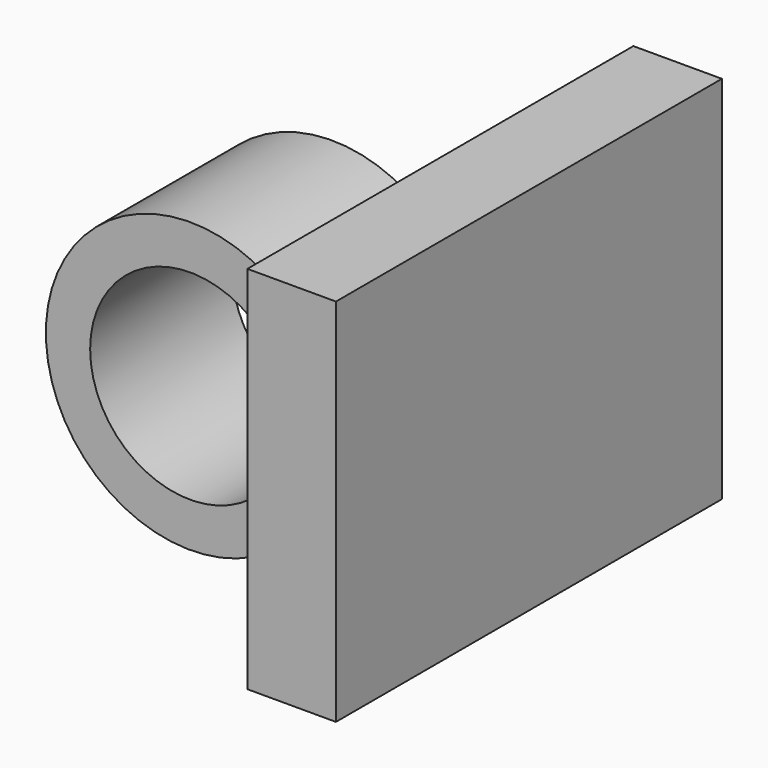
from build123d import *

# Parameters (mm, degrees)
F0_W     = 69.2029632628
F0_H     = 53.0872046947
F1_DEPTH = 12.7
F3_DEPTH = 25.4
F7_DEPTH = 25.4
F8_DEPTH = 37.1620410511
F9_DEPTH = 12.7


# Not quite as in the source:
# - the program builds the solid bodies; features that only make, move or delete a surface that nothing else refers to are left out


with BuildPart() as f1:
    # F0 (on Right) → F1 (new body)
    with BuildSketch(Plane.YZ):
        with Locations((-2.5595594198, -0.3791954368)):
            Rectangle(F0_W, F0_H)
    extrude(amount=F1_DEPTH)


with BuildPart() as f3:
    # F2 (on Front) → F3 (new body)
    with BuildSketch(Plane.XZ):
        with BuildLine():
            Line((0, -10.0486492738), (0, 11.755024083))
            ThreePointArc((0, 11.755024083), (-38.3185949727, 0.8531874046), (0, -10.0486492738))
        make_face()
    extrude(amount=F3_DEPTH)


with BuildPart() as f7:
    # F2 (on Front) → F7 (new body)
    with BuildSketch(Plane.XZ):
        with BuildLine():
            Line((0, -10.0486492738), (0, 11.755024083))
            ThreePointArc((0, 11.755024083), (-38.3185949727, 0.8531874046), (0, -10.0486492738))
        make_face()
    extrude(amount=F7_DEPTH)


with BuildPart() as f8_tool:
    # F4 (on Front) → F8 (new body, through all)
    with BuildSketch(Plane.XZ):
        with BuildLine():
            ThreePointArc((-5.3990000004, -6.7059981609), (-3.2919727747, 0.8531874046), (-5.3990000004, 8.41237297))
            ThreePointArc((-5.3990000004, 8.41237297), (-31.9685935974, 0.8531874046), (-5.3990000004, -6.7059981609))
        make_face()
    extrude(amount=F8_DEPTH)


with BuildPart() as f3_1:
    add(f3.part)

    # F8: cut by f8_tool
    add(f8_tool.part, mode=Mode.SUBTRACT)


with BuildPart() as f7_1:
    add(f7.part)

    # F8: cut by f8_tool
    add(f8_tool.part, mode=Mode.SUBTRACT)


with BuildPart() as f9:
    # F0 (on Right) → F9 (new body)
    with BuildSketch(Plane.YZ):
        with Locations((-2.5595594198, -0.3791954368)):
            Rectangle(F0_W, F0_H)
    extrude(amount=F9_DEPTH)


solid = Compound([f1.part, f3_1.part, f7_1.part, f9.part])
